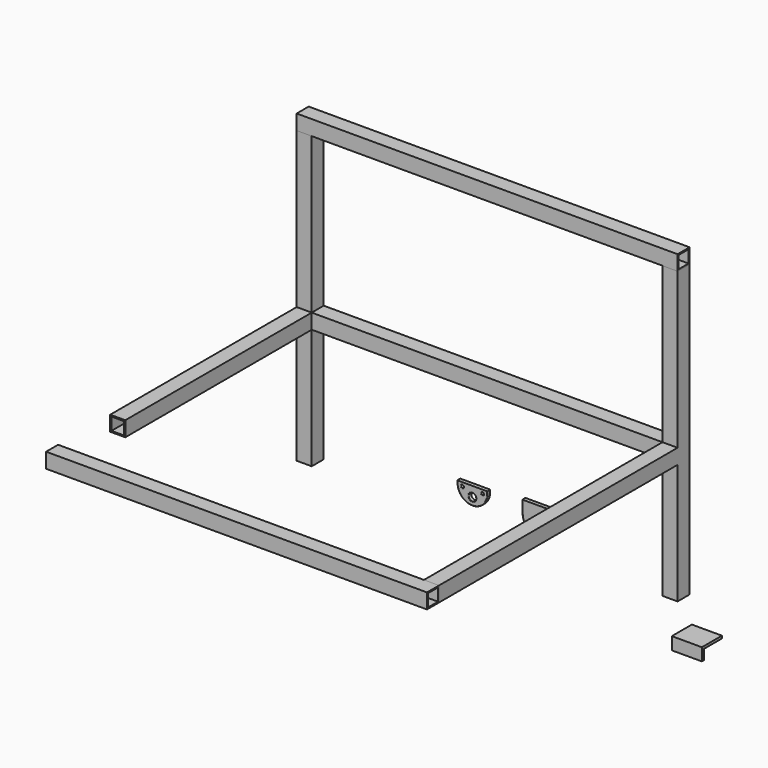
from build123d import *

# Parameters (mm, degrees)
F0_W      = 38.1
F0_H      = 38.1
F0_W_2    = 31.75
F0_H_2    = 31.75
F1_DEPTH  = 342.9
F2_W      = 38.1
F2_H      = 38.1
F2_W_2    = 31.75
F2_H_2    = 31.75
F3_DEPTH  = 889
F4_W      = 38.1
F4_H      = 38.1
F4_W_2    = 31.75
F4_H_2    = 31.75
F5_DEPTH  = 304.8
F6_DEPTH  = 38.1
F7_DEPTH  = 393.7
F8_W      = 38.1
F8_H      = 38.1
F8_W_2    = 31.75
F8_H_2    = 31.75
F9_DEPTH  = 393.7
F10_W     = 38.1
F10_H     = 38.1
F10_W_2   = 31.75
F10_H_2   = 31.75
F11_DEPTH = 965.2
F12_W     = 31.75
F12_H     = 31.75
F13_DEPTH = 590.55
F14_W     = 38.1
F14_H     = 38.1
F14_W_2   = 31.75
F14_H_2   = 31.75
F15_DEPTH = 755.65
F17_DEPTH = 76.2
F18_R     = 9.525
F18_R_2   = 3.37312
F19_DEPTH = 9.525
F20_R     = 1.27
F22_DEPTH = 9.525
F23_R     = 1.27
F24_W     = 38.1
F24_H     = 38.1
F24_W_2   = 31.75
F24_H_2   = 31.75
F25_DEPTH = 965.2


with BuildPart() as f1:
    # F0 (on Top) → F1 (new body)
    with BuildSketch(Plane.XY):
        Rectangle(F0_W, F0_H)
        Rectangle(F0_W_2, F0_H_2, mode=Mode.SUBTRACT)
    extrude(amount=F1_DEPTH)

    # F2 (on face) → F3 (join)
    with BuildSketch(Plane(origin=(-19.05, 0, 0), x_dir=(0, -1, 0), z_dir=(-1, 0, 0))):
        with Locations((0, 323.85)):
            Rectangle(F2_W, F2_H)
        with Locations((0, 323.85)):
            Rectangle(F2_W_2, F2_H_2, mode=Mode.SUBTRACT)
    extrude(amount=F3_DEPTH)

    # F8 (on face) → F9 (join)
    with BuildSketch(Plane.XY.offset(342.9)):
        Rectangle(F8_W, F8_H)
        Rectangle(F8_W_2, F8_H_2, mode=Mode.SUBTRACT)
    extrude(amount=F9_DEPTH)

    # F14 (on face) → F15 (join)
    with BuildSketch(Plane.XZ.offset(19.05)):
        with Locations((0, 323.85)):
            Rectangle(F14_W, F14_H)
        with Locations((0, 323.85)):
            Rectangle(F14_W_2, F14_H_2, mode=Mode.SUBTRACT)
    extrude(amount=F15_DEPTH)


with BuildPart() as f5:
    # F4 (on face) → F5 (new body)
    with BuildSketch(Plane(origin=(0, 0, 304.8), x_dir=(1, 0, 0), z_dir=(0, 0, -1))):
        with Locations((-927.1, 0)):
            Rectangle(F4_W, F4_H)
        with Locations((-927.1, 0)):
            Rectangle(F4_W_2, F4_H_2, mode=Mode.SUBTRACT)
    extrude(amount=F5_DEPTH)


with BuildPart() as f6:
    # F6 (new): a face of the model
    f6_faces = [f5.part.faces().sort_by_distance(p)[0] for p in [
        (-908.5888153673, 0, 304.8),
    ]]
    extrude(f6_faces, amount=F6_DEPTH)

    # F7 (add): a face of the model
    f7_faces = [f6.faces().sort_by_distance(p)[0] for p in [
        (-908.5888153673, 0, 342.9),
    ]]
    extrude(f7_faces, amount=F7_DEPTH)


with BuildPart() as f11:
    # F10 (on face) → F11 (new body)
    with BuildSketch(Plane(origin=(-946.15, 0, 0), x_dir=(0, -1, 0), z_dir=(-1, 0, 0))):
        with Locations((0, 755.65)):
            Rectangle(F10_W, F10_H)
        with Locations((0, 755.65)):
            Rectangle(F10_W_2, F10_H_2, mode=Mode.SUBTRACT)
    extrude(amount=-F11_DEPTH)


with BuildPart() as f13:
    # F12 (on face) → F13 (new body)
    with BuildSketch(Plane.XZ.offset(19.05)):
        Polygon((-908.05, 304.8), (-908.05, 342.9), (-946.15, 342.9), (-946.15, 304.6984), (-908.05, 304.6984), align=None)
        with Locations((-927.1, 323.7484)):
            Rectangle(F12_W, F12_H, mode=Mode.SUBTRACT)
    extrude(amount=F13_DEPTH)


with BuildPart() as f17:
    # F16 (on Right) → F17 (new body)
    with BuildSketch(Plane.YZ):
        Polygon((50.0031399928, -92.0927183867), (50.0031399928, -85.7427183867), (-13.4968600072, -85.7427183867), (-13.4968600072, -117.4927183867), (-7.1468600072, -117.4927183867), (-7.1468600072, -92.0927183867), align=None)
    extrude(amount=F17_DEPTH)


with BuildPart() as f19:
    # F18 (on Front) → F19 (new body)
    with BuildSketch(Plane.XZ):
        with BuildLine():
            Line((-546.7213775635, 82.477462914), (-546.7213775635, 76.127462914))
            ThreePointArc((-546.7213775635, 76.127462914), (-508.6213775635, 38.027462914), (-470.5213775635, 76.127462914))
            Line((-470.5213775635, 76.127462914), (-470.5213775635, 82.477462914))
            Line((-470.5213775635, 82.477462914), (-483.2213775635, 82.477462914))
            Line((-483.2213775635, 82.477462914), (-546.7213775635, 82.477462914))
        make_face()
        with Locations((-508.8159826909, 57.0784569335)):
            Circle(F18_R, mode=Mode.SUBTRACT)
        with Locations((-534.0213775635, 72.754342914)):
            Circle(F18_R_2, mode=Mode.SUBTRACT)
        with BuildLine():
            ThreePointArc((-479.8482575635, 72.952462914), (-485.6065335892, 70.5673068883), (-483.2213775635, 76.325582914))
            ThreePointArc((-483.2213775635, 76.325582914), (-480.8362215377, 75.3376189398), (-479.8482575635, 72.952462914))
        make_face(mode=Mode.SUBTRACT)
    extrude(amount=F19_DEPTH)

    # F20
    f20_edges = [f19.edges().sort_by_distance(p)[0] for p in [
        (-537.394498, -9.525, 72.754343),
        (-518.340983, -9.525, 57.078457),
        (-483.221378, -9.525, 69.579343),
        (-508.621378, -9.525, 38.027463),
        (-483.221378, 0, 69.579343),
        (-537.394498, 0, 72.754343),
        (-518.340983, 0, 57.078457),
        (-508.621378, 0, 38.027463),
    ]]
    fillet(f20_edges, radius=F20_R)


with BuildPart() as f22:
    # F21 (on face) → F22 (new body)
    with BuildSketch(Plane.XZ.offset(9.525)):
        with BuildLine():
            Line((-374.1299766064, 99.3961830735), (-374.1299766064, 67.6461830735))
            ThreePointArc((-374.1299766064, 67.6461830735), (-362.9707449696, 40.7054147103), (-336.0299766064, 29.5461830735))
            ThreePointArc((-336.0299766064, 29.5461830735), (-309.0892082432, 40.7054147103), (-297.9299766064, 67.6461830735))
            Line((-297.9299766064, 67.6461830735), (-297.9299766064, 99.3961830735))
            Line((-297.9299766064, 99.3961830735), (-374.1299766064, 99.3961830735))
        make_face()
        with BuildLine():
            ThreePointArc((-326.5049766064, 48.5961830735), (-329.2947845156, 41.8609909827), (-336.0299766064, 39.0711830735))
            ThreePointArc((-336.0299766064, 39.0711830735), (-342.7651686972, 55.3313751643), (-326.5049766064, 48.5961830735))
        make_face(mode=Mode.SUBTRACT)
    extrude(amount=F22_DEPTH)

    # F23
    f23_edges = [f22.edges().sort_by_distance(p)[0] for p in [
        (-345.554977, -19.05, 48.596183),
        (-336.029977, -19.05, 29.546183),
        (-297.929977, -19.05, 83.521183),
        (-374.129977, -19.05, 83.521183),
        (-345.554977, -9.525, 48.596183),
        (-336.029977, -9.525, 29.546183),
        (-297.929977, -9.525, 83.521183),
        (-374.129977, -9.525, 83.521183),
    ]]
    fillet(f23_edges, radius=F23_R)


with BuildPart() as f25:
    # F24 (on face) → F25 (new body)
    with BuildSketch(Plane.YZ.offset(19.05)):
        with Locations((-793.75, 323.85)):
            Rectangle(F24_W, F24_H)
        with Locations((-793.75, 323.85)):
            Rectangle(F24_W_2, F24_H_2, mode=Mode.SUBTRACT)
    extrude(amount=-F25_DEPTH)


solid = Compound([f1.part, f5.part, f6.part, f11.part, f13.part, f17.part, f19.part, f22.part, f25.part])
